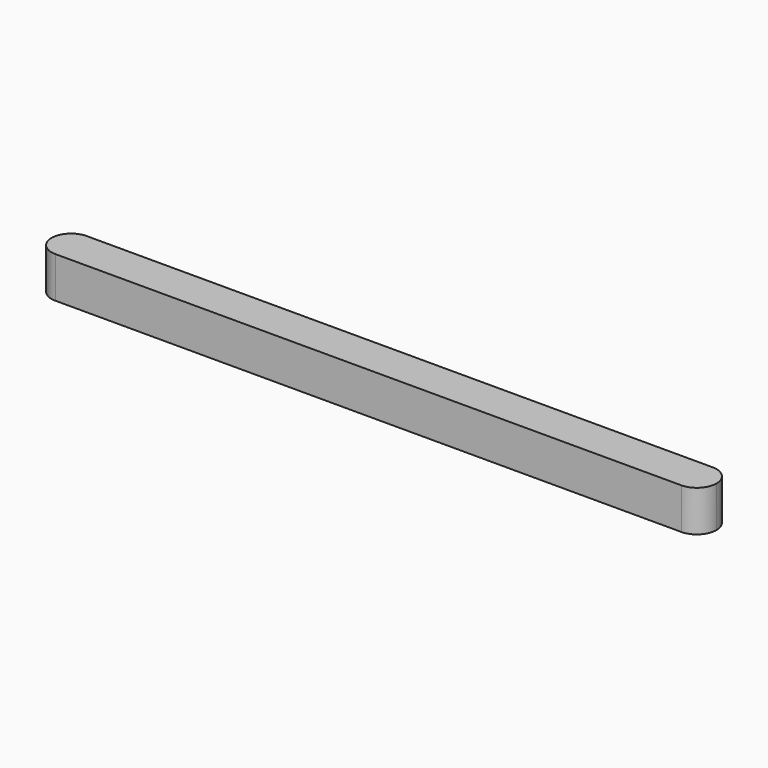
from build123d import *

# Parameters (mm, degrees)
F0_W     = 34
F0_H     = 2
F1_DEPTH = 2.1
F2_R     = 0.99999


# Not quite as in the source:
# - a fillet or chamfer is up to 0.001 mm smaller than in the source, because OpenCascade refuses the exact size


with BuildPart() as f1:
    # F0 (on Top) → F1 (new body)
    with BuildSketch(Plane.XY):
        Rectangle(F0_W, F0_H)
    extrude(amount=F1_DEPTH)

    # F2 (radius 1 in the source; OpenCascade refuses exactly that, so slightly less here)
    f2_edges = [f1.edges().sort_by_distance(p)[0] for p in [
        (17, 1, 1.05),
        (17, -1, 1.05),
        (-17, -1, 1.05),
        (-17, 1, 1.05),
    ]]
    fillet(f2_edges, radius=F2_R)


solid = f1.part
